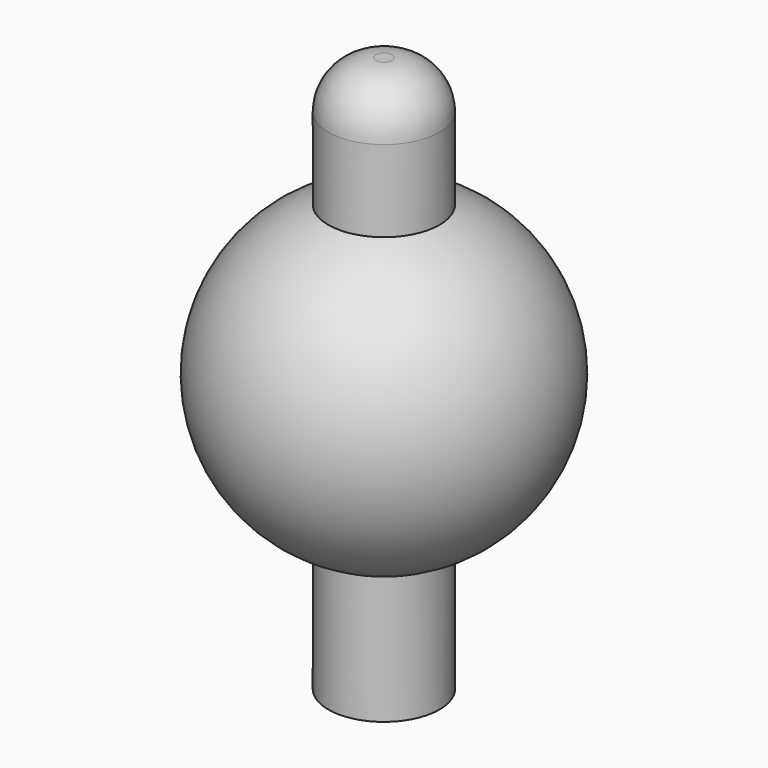
from build123d import *

# Parameters (mm, degrees)
F0_R     = 7
F0_R_2   = 5
F0_R_3   = 3.75
F1_DEPTH = 70
F4_DEPTH = 35
F5_R     = 6


with BuildPart() as f1:
    # F0 (on Top) → F1 (new body)
    with BuildSketch(Plane.XY):
        Circle(F0_R)
        Circle(F0_R_2, mode=Mode.SUBTRACT)
        Circle(F0_R_2)
        Circle(F0_R_3, mode=Mode.SUBTRACT)
        Circle(F0_R_3)
    extrude(amount=F1_DEPTH)

    # F2 (on Front) → F3 (revolve)
    with BuildSketch(Plane.XZ):
        with BuildLine():
            ThreePointArc((0, 55), (-20, 35), (0, 15))
            Line((0, 15), (0, 55))
        make_face()
    revolve(axis=Axis((0, 0, 35), (0, 0, 1)))

    # F0 (on Top) → F4 (cut)
    with BuildSketch(Plane.XY):
        Circle(F0_R_2)
        Circle(F0_R_3, mode=Mode.SUBTRACT)
    extrude(amount=F4_DEPTH, mode=Mode.SUBTRACT)

    # F5
    f5_edges = [f1.edges().sort_by_distance(p)[0] for p in [
        (-7, 0, 70),
    ]]
    fillet(f5_edges, radius=F5_R)


solid = f1.part
